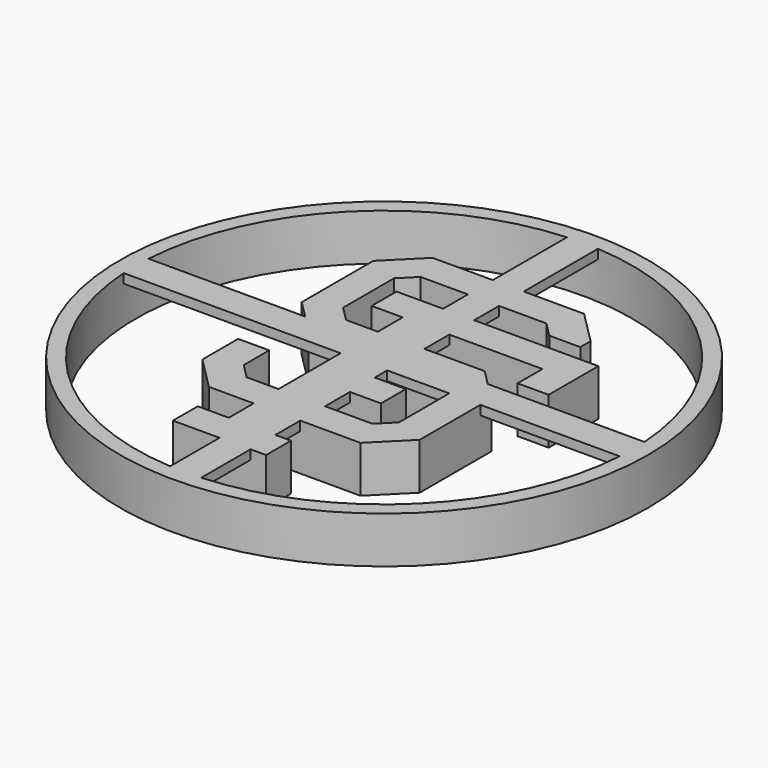
from build123d import *

# Parameters (mm, degrees)
F4_DEPTH = 15
F5_R     = 85
F5_R_2   = 80
F6_DEPTH = 15
F7_W     = 10
F7_H     = 10
F8_DEPTH = 3


with BuildPart() as f4:
    # F3 (on Top) → F4 (new body)
    with BuildSketch(Plane.XY):
        Polygon((24.3933982822, 50), (-24.3933982822, 50), (-35, 39.3933982822), (-35, 10.6066017178), (-24.3933982822, 0), (-10, 0), (-10, -30), (-20.2512626585, -30), (-25, -25.2512626585), (-25, -15), (-35, -15), (-35, -29.3933982822), (-24.3933982822, -40), (-10, -40), (-10, -50), (-20, -50), (-20, -60), (10, -60), (10, -50), (0, -50), (0, -40), (24.3933982822, -40), (35, -29.3933982822), (35, -0.6066017178), (24.3933982822, 10), (0, 10), (0, 12.3223304703), (0, 20), (35, 20), (35, 10), (45, 10), (45, 30), (-20, 30), (-20, 20), (-10, 20), (-10, 18.4070525334), (-10, 10), (-20.2512626585, 10), (-25, 14.7487373415), (-25, 18.8908729653), (-25, 35.2512626585), (-20.2512626585, 40), (20.2512626585, 40), (25, 35.2512626585), (35, 35.2512626585), (35, 39.3933982822), align=None)
        Polygon((20.2512626585, 0), (25, -4.7487373415), (25, -25.2512626585), (20.2512626585, -30), (0, -30), (0, -20), (15, -20), (15, -10), (0, -10), (0, 0), align=None, mode=Mode.SUBTRACT)
    extrude(amount=F4_DEPTH)



with BuildPart() as f6:
    # F5 (on Top) → F6 (new body)
    with BuildSketch(Plane.XY):
        Circle(F5_R)
        Circle(F5_R_2, mode=Mode.SUBTRACT)
    extrude(amount=F6_DEPTH)


with BuildPart() as f4_1:
    add(f4.part)

    add(f6.part)  # F8 merges F6
    # F7 (on face) → F8 (join)
    with BuildSketch(Plane.XY.offset(15)):
        Rectangle(F7_W, F7_H)
        with BuildLine():
            Line((79.8435971134, 5), (5, 5))
            Line((5, 5), (5, -5))
            Line((5, -5), (79.8435971134, -5))
            ThreePointArc((79.8435971134, -5), (79.9608897183, -2.5012227941), (80, 0))
            ThreePointArc((80, 0), (79.9608897183, 2.5012227941), (79.8435971134, 5))
        make_face()
        with BuildLine():
            Line((-5, 79.8435971134), (-5, 5))
            Line((-5, 5), (5, 5))
            Line((5, 5), (5, 79.8435971134))
            ThreePointArc((5, 79.8435971134), (0, 80), (-5, 79.8435971134))
        make_face()
        with BuildLine():
            Line((-5, 5), (-79.8435971134, 5))
            ThreePointArc((-79.8435971134, 5), (-80, 0), (-79.8435971134, -5))
            Line((-79.8435971134, -5), (-5, -5))
            Line((-5, -5), (-5, 5))
        make_face()
        with BuildLine():
            Line((5, -5), (-5, -5))
            Line((-5, -5), (-5, -79.8435971134))
            ThreePointArc((-5, -79.8435971134), (0, -80), (5, -79.8435971134))
            Line((5, -79.8435971134), (5, -5))
        make_face()
    extrude(amount=-F8_DEPTH)


solid = f4_1.part
